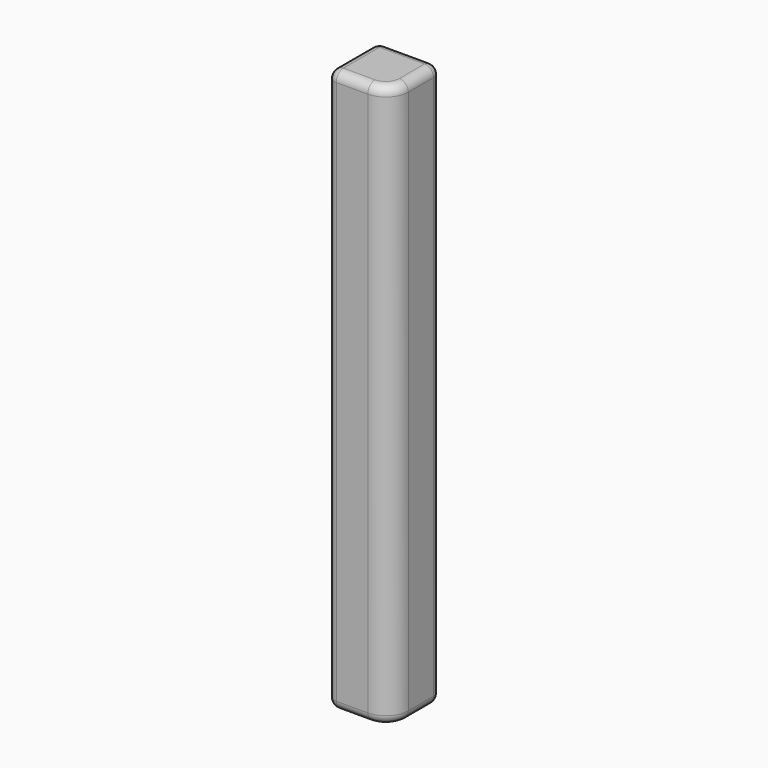
from build123d import *

# Parameters (mm, degrees)
F0_W         = 14
F0_H         = 14
F1_DEPTH     = 125
F2_R         = 2
F3_T1_DEPTH  = 125
F3_T4_ANGLE  = 90
F3_T6_ANGLE  = 90
F4_T1_DEPTH  = 121
F4_T3_DEPTH  = 10
F4_S7_W      = 2
F4_S7_H      = 2
F4_T8_DEPTH  = 2
F4_S13_W     = 2
F4_S13_H     = 2
F4_T14_DEPTH = 2
F4_T18_ANGLE = 90


# Not quite as in the source:
# - a fillet or chamfer that OpenCascade refuses, or shapes differently, is made with other operations: its cross-section is extruded or revolved along the edge and cut away or added


with BuildPart() as f1:
    # F0 (on Top) → F1 (new body)
    with BuildSketch(Plane.XY):
        with Locations((-7, -7)):
            Rectangle(F0_W, F0_H)
    extrude(amount=F1_DEPTH)

    # F2
    f2_edges = [f1.edges().sort_by_distance(p)[0] for p in [
        (-7, -14, 125),
        (0, -7, 125),
        (-7, -14, 0),
        (0, -7, 0),
        (-14, -7, 125),
        (-7, 0, 125),
        (-14, 0, 62.5),
        (-14, -14, 62.5),
        (-14, -7, 0),
    ]]
    fillet(f2_edges, radius=F2_R)

    # F3: fillet of radius 5 on 1 edges, made by hand

    # F3_s2 → F3_t1 (cut)
    with BuildSketch(Plane.XY):
        with BuildLine():
            ThreePointArc((0, -9), (-1.4644660941, -12.5355339059), (-5, -14))
            Line((-5, -14), (0, -14))
            Line((0, -14), (0, -9))
        make_face()
    extrude(amount=F3_T1_DEPTH, mode=Mode.SUBTRACT)

    # F3_s3 → F3_t4 (revolve, cut)
    with BuildSketch(Plane.XZ.offset(9)):
        with BuildLine():
            ThreePointArc((-2, 0), (-0.5857864376, 0.5857864376), (0, 2))
            Line((0, 2), (0, 0))
            Line((0, 0), (-2, 0))
        make_face()
    revolve(axis=Axis((-5, -9, 0), (0, 0, -1)), revolution_arc=F3_T4_ANGLE, mode=Mode.SUBTRACT)

    # F3_s5 → F3_t6 (revolve, cut)
    with BuildSketch(Plane.YZ.offset(-5)):
        with BuildLine():
            ThreePointArc((-12, 125), (-13.4142135624, 124.4142135624), (-14, 123))
            Line((-14, 123), (-14, 125))
            Line((-14, 125), (-12, 125))
        make_face()
    revolve(axis=Axis((-5, -9, 125), (0, 0, 1)), revolution_arc=F3_T6_ANGLE, mode=Mode.SUBTRACT)

    # F4: fillet of radius 2 on 2 edges, made by hand

    # F4_s2 → F4_t1 (cut)
    with BuildSketch(Plane.XY.offset(2)):
        with BuildLine():
            ThreePointArc((0, -2), (-0.5857864376, -0.5857864376), (-2, 0))
            Line((-2, 0), (0, 0))
            Line((0, 0), (0, -2))
        make_face()
    extrude(amount=F4_T1_DEPTH, mode=Mode.SUBTRACT)

    # F4_s4 → F4_t3 (cut)
    with BuildSketch(Plane.YZ.offset(-12)):
        with BuildLine():
            ThreePointArc((0, 2), (-0.5857864376, 0.5857864376), (-2, 0))
            Line((-2, 0), (0, 0))
            Line((0, 0), (0, 2))
        make_face()
    extrude(amount=F4_T3_DEPTH, mode=Mode.SUBTRACT)


with BuildPart() as f4_tool6:
    # F4_s7 → F4_t8 (new body)
    with BuildSketch(Plane.YZ.offset(-2)):
        with Locations((-1, 124)):
            Rectangle(F4_S7_W, F4_S7_H)
    extrude(amount=F4_T8_DEPTH)

    # F4_s9 → F4_t10 (revolve, cut)
    with BuildSketch(Plane(origin=(-2, -2, 123), x_dir=(0, -0.7071067812, -0.7071067812), z_dir=(0, -0.7071067812, 0.7071067812))):
        with BuildLine():
            ThreePointArc((0, -2), (2, 0), (0, 2))
            Line((0, 2), (0, -2))
        make_face()
    revolve(axis=Axis((-2, -2, 123), (1, 0, 0)), mode=Mode.SUBTRACT)


with BuildPart() as f1_1:
    add(f1.part)

    # F4_t5: cut F4_tool6
    add(f4_tool6.part, mode=Mode.SUBTRACT)


with BuildPart() as f4_tool12:
    # F4_s13 → F4_t14 (new body)
    with BuildSketch(Plane.XZ.offset(2)):
        with Locations((-13, 1)):
            Rectangle(F4_S13_W, F4_S13_H)
    extrude(amount=-F4_T14_DEPTH)

    # F4_s15 → F4_t16 (revolve, cut)
    with BuildSketch(Plane(origin=(-12, -2, 2), x_dir=(0.7071067812, 0, 0.7071067812), z_dir=(-0.7071067812, 0, 0.7071067812))):
        with BuildLine():
            ThreePointArc((0, -2), (2, 0), (0, 2))
            Line((0, 2), (0, -2))
        make_face()
    revolve(axis=Axis((-12, -2, 2), (0, 1, 0)), mode=Mode.SUBTRACT)


with BuildPart() as f1_2:
    add(f1_1.part)

    # F4_t11: cut F4_tool12
    add(f4_tool12.part, mode=Mode.SUBTRACT)

    # F4_s17 → F4_t18 (revolve, cut)
    with BuildSketch(Plane.XY.offset(2)):
        with BuildLine():
            ThreePointArc((0, -2), (-0.5857864376, -0.5857864376), (-2, 0))
            Line((-2, 0), (0, 0))
            Line((0, 0), (0, -2))
        make_face()
    revolve(axis=Axis((-2, 0, 2), (0, 1, 0)), revolution_arc=F4_T18_ANGLE, mode=Mode.SUBTRACT)


solid = f1_2.part
